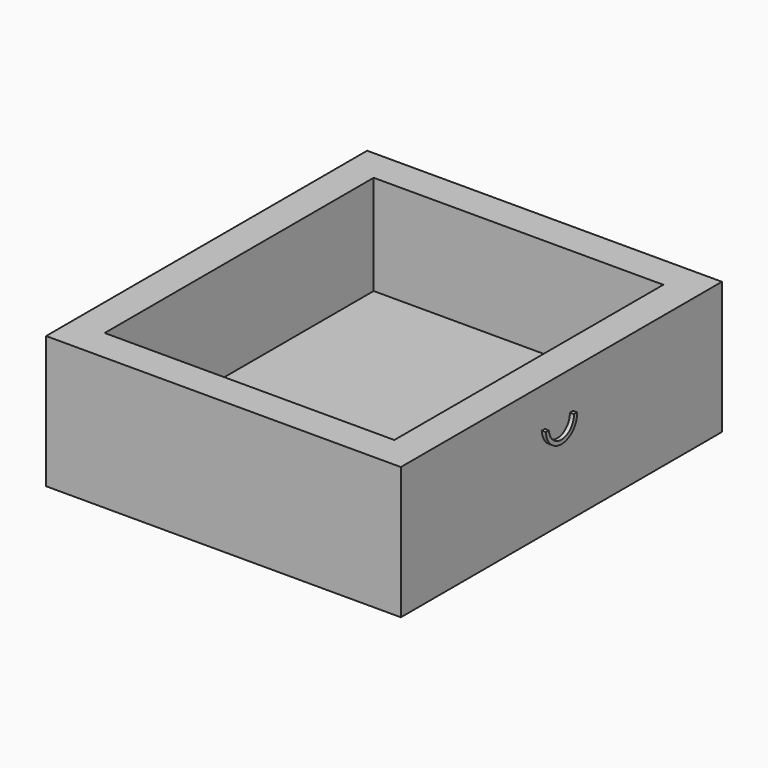
from build123d import *

# Parameters (mm, degrees)
F0_W     = 346
F0_H     = 129
F1_DEPTH = 195.7
F2_W     = 282.5
F2_H     = 327.9
F3_DEPTH = 97.25
F5_DEPTH = 4


# Not quite as in the source:
# - a feature names something its author has since deleted; it is built from what else it names


with BuildPart() as f1:
    # F0 (on Front) → F1 (new body, symmetric)
    with BuildSketch(Plane.XZ):
        Rectangle(F0_W, F0_H)
    extrude(amount=F1_DEPTH, both=True)

    # F2 (on face) → F3 (cut)
    with BuildSketch(Plane.XY.offset(64.5)):
        Rectangle(F2_W, F2_H)
    extrude(amount=-F3_DEPTH, mode=Mode.SUBTRACT)

    # F4 (on face) → F5 (join)
    with BuildSketch(Plane.YZ.offset(173)):
        with BuildLine():
            Line((-20.1823599637, 25.9178485721), (-23.953853175, 25.9178485721))
            ThreePointArc((-23.953853175, 25.9178485721), (-4.0838683271, 7.9147781718), (14.2255900428, 27.5027994066))
            Line((14.2255900428, 27.5027994066), (10.32506302, 27.5027994066))
            ThreePointArc((10.32506302, 27.5027994066), (-4.1526228185, 11.7732405564), (-20.1823599637, 25.9178485721))
        make_face()
    extrude(amount=F5_DEPTH)


solid = f1.part
